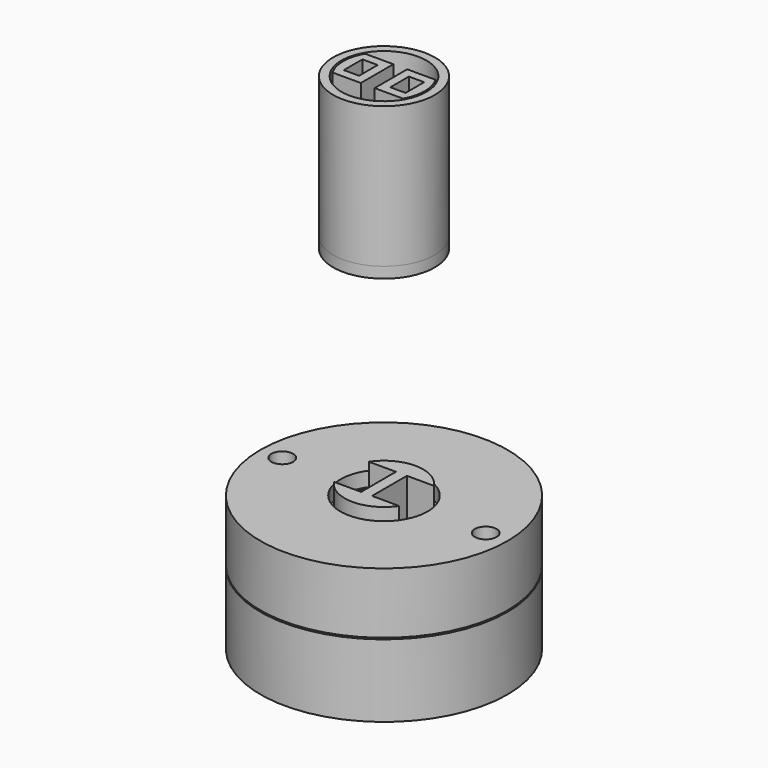
from build123d import *

# Parameters (mm, degrees)
F5_R      = 17
F5_W      = 21.213204
F5_H      = 21.213204
F5_R_2    = 8.1
F5_R_3    = 6
F6_DEPTH  = 0.5
F7_DEPTH  = 10
F8_W      = 20.78894
F8_H      = 20.78894
F8_R      = 6
F8_W_2    = 1.5
F8_H_2    = 8
F9_DEPTH  = 0.9
F10_W     = 20.364676
F10_H     = 20.364676
F10_R     = 8.1
F11_DEPTH = 8.6
F12_R     = 1.1
F12_R_2   = 1
F14_W     = 2
F14_H     = 15
F18_R     = 17
F18_W     = 21.213204
F18_H     = 21.213204
F18_R_2   = 8.2
F18_R_3   = 6
F19_DEPTH = 2
F20_DEPTH = 6.4
F21_R     = 1.5
F22_DEPTH = 18.6
F25_DEPTH = 18.4
F27_W     = 2.1
F27_H     = 3.2
F28_DEPTH = 1
F29_DEPTH = 19.4
F30_R     = 7
F30_R_2   = 5.85
F30_R_3   = 4
F31_DEPTH = 1.5
F32_DEPTH = 19.4
F34_DEPTH = 0.9


with BuildPart() as f6:
    # F5 (on Top) → F6 (new body)
    with BuildSketch(Plane.XY):
        Circle(F5_R)
        with BuildLine():
            ThreePointArc((10.606602, 10.606602), (13.858193, 5.740251), (15, 0))
            ThreePointArc((15, 0), (13.858193, -5.740251), (10.606602, -10.606602))
            ThreePointArc((10.606602, -10.606602), (0, -15), (-10.606602, -10.606602))
            ThreePointArc((-10.606602, -10.606602), (-15, 0), (-10.606602, 10.606602))
            ThreePointArc((-10.606602, 10.606602), (0, 15), (10.606602, 10.606602))
        make_face(mode=Mode.SUBTRACT)
        with BuildLine():
            Line((-10.606602, 10.606602), (10.606602, 10.606602))
            ThreePointArc((10.606602, 10.606602), (0, 15), (-10.606602, 10.606602))
        make_face()
        with BuildLine():
            Line((-10.606602, -10.606602), (-10.606602, 10.606602))
            ThreePointArc((-10.606602, 10.606602), (-15, 0), (-10.606602, -10.606602))
        make_face()
        with BuildLine():
            ThreePointArc((10.606602, -10.606602), (13.858193, -5.740251), (15, 0))
            ThreePointArc((15, 0), (13.858193, 5.740251), (10.606602, 10.606602))
            Line((10.606602, 10.606602), (10.606602, -10.606602))
        make_face()
        with BuildLine():
            ThreePointArc((-10.606602, -10.606602), (0, -15), (10.606602, -10.606602))
            Line((10.606602, -10.606602), (-10.606602, -10.606602))
        make_face()
        Rectangle(F5_W, F5_H)
        Circle(F5_R_2, mode=Mode.SUBTRACT)
        Circle(F5_R_2)
        Circle(F5_R_3, mode=Mode.SUBTRACT)
    extrude(amount=F6_DEPTH)

    # F5 (on Top) → F7 (join)
    with BuildSketch(Plane.XY):
        Circle(F5_R)
        with BuildLine():
            ThreePointArc((10.606602, 10.606602), (13.858193, 5.740251), (15, 0))
            ThreePointArc((15, 0), (13.858193, -5.740251), (10.606602, -10.606602))
            ThreePointArc((10.606602, -10.606602), (0, -15), (-10.606602, -10.606602))
            ThreePointArc((-10.606602, -10.606602), (-15, 0), (-10.606602, 10.606602))
            ThreePointArc((-10.606602, 10.606602), (0, 15), (10.606602, 10.606602))
        make_face(mode=Mode.SUBTRACT)
        with BuildLine():
            Line((-10.606602, -10.606602), (-10.606602, 10.606602))
            ThreePointArc((-10.606602, 10.606602), (-15, 0), (-10.606602, -10.606602))
        make_face()
        with BuildLine():
            Line((-10.606602, 10.606602), (10.606602, 10.606602))
            ThreePointArc((10.606602, 10.606602), (0, 15), (-10.606602, 10.606602))
        make_face()
        with BuildLine():
            ThreePointArc((10.606602, -10.606602), (13.858193, -5.740251), (15, 0))
            ThreePointArc((15, 0), (13.858193, 5.740251), (10.606602, 10.606602))
            Line((10.606602, 10.606602), (10.606602, -10.606602))
        make_face()
        with BuildLine():
            ThreePointArc((-10.606602, -10.606602), (0, -15), (10.606602, -10.606602))
            Line((10.606602, -10.606602), (-10.606602, -10.606602))
        make_face()
    extrude(amount=F7_DEPTH)


with BuildPart() as f9:
    # F8 (on face) → F9 (new body)
    with BuildSketch(Plane.XY.offset(0.5)):
        Rectangle(F8_W, F8_H)
        Circle(F8_R, mode=Mode.SUBTRACT)
        Circle(F8_R)
        Rectangle(F8_W_2, F8_H_2, mode=Mode.SUBTRACT)
    extrude(amount=F9_DEPTH)


with BuildPart() as f11:
    # F10 (on face) → F11 (new body)
    with BuildSketch(Plane.XY.offset(1.4)):
        Rectangle(F10_W, F10_H)
        Circle(F10_R, mode=Mode.SUBTRACT)
    extrude(amount=F11_DEPTH)

    # F12 (on Front) → F13 (revolve, cut)
    with BuildSketch(Plane.XZ):
        with Locations((8.5, 7.44)):
            Circle(F12_R)
        with Locations((8.5, 7.44)):
            Circle(F12_R_2, mode=Mode.SUBTRACT)
        with Locations((8.5, 4)):
            Circle(F12_R)
        with Locations((8.5, 4)):
            Circle(F12_R_2, mode=Mode.SUBTRACT)
        with Locations((8.5, 7.44)):
            Circle(F12_R_2)
        with Locations((8.5, 4)):
            Circle(F12_R_2)
    revolve(axis=Axis((0, 0, 11.757353), (0, 0, -1)), mode=Mode.SUBTRACT)


with BuildPart() as f15:
    # F14 (on Front) → F15 (revolve)
    with BuildSketch(Plane.XZ):
        with Locations((6.6, 9.1)):
            Rectangle(F14_W, F14_H)
    revolve(axis=Axis((0, 0, 5.77183), (0, 0, 1)))


with BuildPart() as f16:
    # F12 (on Front) → F16 (revolve)
    with BuildSketch(Plane.XZ):
        with Locations((8.5, 7.44)):
            Circle(F12_R_2)
    revolve(axis=Axis((0, 0, 11.757353), (0, 0, -1)))


with BuildPart() as f16b:
    # F12 (on Front) → F16, piece 2 (revolve)
    with BuildSketch(Plane.XZ):
        with Locations((8.5, 4)):
            Circle(F12_R_2)
    revolve(axis=Axis((0, 0, 11.757353), (0, 0, -1)))


with BuildPart() as f19:
    # F18 (on offset) → F19 (new body)
    with BuildSketch(Plane.XY.offset(16.6)):
        Circle(F18_R)
        with BuildLine():
            ThreePointArc((10.606602, 10.606602), (13.858193, 5.740251), (15, 0))
            ThreePointArc((15, 0), (13.858193, -5.740251), (10.606602, -10.606602))
            ThreePointArc((10.606602, -10.606602), (0, -15), (-10.606602, -10.606602))
            ThreePointArc((-10.606602, -10.606602), (-15, 0), (-10.606602, 10.606602))
            ThreePointArc((-10.606602, 10.606602), (0, 15), (10.606602, 10.606602))
        make_face(mode=Mode.SUBTRACT)
        Rectangle(F18_W, F18_H)
        Circle(F18_R_2, mode=Mode.SUBTRACT)
        Circle(F18_R_2)
        Circle(F18_R_3, mode=Mode.SUBTRACT)
        with BuildLine():
            Line((-10.606602, 10.606602), (10.606602, 10.606602))
            ThreePointArc((10.606602, 10.606602), (0, 15), (-10.606602, 10.606602))
        make_face()
        with BuildLine():
            Line((-10.606602, -10.606602), (-10.606602, 10.606602))
            ThreePointArc((-10.606602, 10.606602), (-15, 0), (-10.606602, -10.606602))
        make_face()
        with BuildLine():
            ThreePointArc((-10.606602, -10.606602), (0, -15), (10.606602, -10.606602))
            Line((10.606602, -10.606602), (-10.606602, -10.606602))
        make_face()
        with BuildLine():
            ThreePointArc((10.606602, -10.606602), (13.858193, -5.740251), (15, 0))
            ThreePointArc((15, 0), (13.858193, 5.740251), (10.606602, 10.606602))
            Line((10.606602, 10.606602), (10.606602, -10.606602))
        make_face()
    extrude(amount=F19_DEPTH)

    # F18 (on offset) → F20 (join)
    with BuildSketch(Plane.XY.offset(16.6)):
        Circle(F18_R)
        with BuildLine():
            ThreePointArc((10.606602, 10.606602), (13.858193, 5.740251), (15, 0))
            ThreePointArc((15, 0), (13.858193, -5.740251), (10.606602, -10.606602))
            ThreePointArc((10.606602, -10.606602), (0, -15), (-10.606602, -10.606602))
            ThreePointArc((-10.606602, -10.606602), (-15, 0), (-10.606602, 10.606602))
            ThreePointArc((-10.606602, 10.606602), (0, 15), (10.606602, 10.606602))
        make_face(mode=Mode.SUBTRACT)
        with BuildLine():
            ThreePointArc((-10.606602, -10.606602), (0, -15), (10.606602, -10.606602))
            Line((10.606602, -10.606602), (-10.606602, -10.606602))
        make_face()
        with BuildLine():
            Line((-10.606602, -10.606602), (-10.606602, 10.606602))
            ThreePointArc((-10.606602, 10.606602), (-15, 0), (-10.606602, -10.606602))
        make_face()
        with BuildLine():
            ThreePointArc((10.606602, -10.606602), (13.858193, -5.740251), (15, 0))
            ThreePointArc((15, 0), (13.858193, 5.740251), (10.606602, 10.606602))
            Line((10.606602, 10.606602), (10.606602, -10.606602))
        make_face()
        with BuildLine():
            Line((-10.606602, 10.606602), (10.606602, 10.606602))
            ThreePointArc((10.606602, 10.606602), (0, 15), (-10.606602, 10.606602))
        make_face()
    extrude(amount=-F20_DEPTH)


with BuildPart() as f22_tool:
    # F21 (on face) → F22 (new body, through all)
    with BuildSketch(Plane.XY.offset(18.6)):
        with Locations((-14, 0)):
            Circle(F21_R)
        with Locations((14, 0)):
            Circle(F21_R)
    extrude(amount=-F22_DEPTH)


with BuildPart() as f6_1:
    add(f6.part)

    # F22: cut by f22_tool
    add(f22_tool.part, mode=Mode.SUBTRACT)


with BuildPart() as f19_1:
    add(f19.part)

    # F22: cut by f22_tool
    add(f22_tool.part, mode=Mode.SUBTRACT)


with BuildPart() as f25:
    # F24 (on offset) → F25 (new body, through all)
    with BuildSketch(Plane.XY.offset(20)):
        with BuildLine():
            Line((-0.75, -3), (-4.489989, -3))
            ThreePointArc((-4.489989, -3), (0, -5.4), (4.489989, -3))
            Line((4.489989, -3), (0.75, -3))
            Line((0.75, -3), (0.75, 0))
            Line((0.75, 0), (0.75, 3))
            Line((0.75, 3), (4.489989, 3))
            ThreePointArc((4.489989, 3), (0, 5.4), (-4.489989, 3))
            Line((-4.489989, 3), (-0.75, 3))
            Line((-0.75, 3), (-0.75, 0))
            Line((-0.75, 0), (-0.75, -3))
        make_face()
    extrude(amount=-F25_DEPTH)


with BuildPart() as f28:
    # F27 (on offset) → F28 (new body)
    with BuildSketch(Plane.XY.offset(50)):
        with BuildLine():
            Line((0.95, 2.8), (4.849742, 2.8))
            ThreePointArc((4.849742, 2.8), (0, 5.6), (-4.849742, 2.8))
            Line((-4.849742, 2.8), (-0.95, 2.8))
            Line((-0.95, 2.8), (-0.95, -2.8))
            Line((-0.95, -2.8), (-4.849742, -2.8))
            ThreePointArc((-4.849742, -2.8), (0, -5.6), (4.849742, -2.8))
            Line((4.849742, -2.8), (0.95, -2.8))
            Line((0.95, -2.8), (0.95, 2.8))
        make_face()
        with BuildLine():
            ThreePointArc((4.849742, -2.8), (5.409185, -1.449387), (5.6, 0))
            ThreePointArc((5.6, 0), (5.409185, 1.449387), (4.849742, 2.8))
            Line((4.849742, 2.8), (0.95, 2.8))
            Line((0.95, 2.8), (0.95, -2.8))
            Line((0.95, -2.8), (4.849742, -2.8))
        make_face()
        with Locations((3.2, 0)):
            Rectangle(F27_W, F27_H, mode=Mode.SUBTRACT)
        with BuildLine():
            Line((-0.95, 2.8), (-4.849742, 2.8))
            ThreePointArc((-4.849742, 2.8), (-5.6, 0), (-4.849742, -2.8))
            Line((-4.849742, -2.8), (-0.95, -2.8))
            Line((-0.95, -2.8), (-0.95, 2.8))
        make_face()
        with Locations((-3.2, 0)):
            Rectangle(F27_W, F27_H, mode=Mode.SUBTRACT)
        with Locations((3.2, 0)):
            Rectangle(F27_W, F27_H)
        with Locations((-3.2, 0)):
            Rectangle(F27_W, F27_H)
    extrude(amount=F28_DEPTH)

    # F27 (on offset) → F29 (join)
    with BuildSketch(Plane.XY.offset(50)):
        with BuildLine():
            Line((-0.95, 2.8), (-4.849742, 2.8))
            ThreePointArc((-4.849742, 2.8), (-5.6, 0), (-4.849742, -2.8))
            Line((-4.849742, -2.8), (-0.95, -2.8))
            Line((-0.95, -2.8), (-0.95, 2.8))
        make_face()
        with Locations((-3.2, 0)):
            Rectangle(F27_W, F27_H, mode=Mode.SUBTRACT)
        with BuildLine():
            ThreePointArc((4.849742, -2.8), (5.409185, -1.449387), (5.6, 0))
            ThreePointArc((5.6, 0), (5.409185, 1.449387), (4.849742, 2.8))
            Line((4.849742, 2.8), (0.95, 2.8))
            Line((0.95, 2.8), (0.95, -2.8))
            Line((0.95, -2.8), (4.849742, -2.8))
        make_face()
        with Locations((3.2, 0)):
            Rectangle(F27_W, F27_H, mode=Mode.SUBTRACT)
    extrude(amount=F29_DEPTH)


with BuildPart() as f31:
    # F30 (on offset) → F31 (new body)
    with BuildSketch(Plane.XY.offset(50)):
        Circle(F30_R)
        Circle(F30_R_2, mode=Mode.SUBTRACT)
        Circle(F30_R_2)
        Circle(F30_R_3, mode=Mode.SUBTRACT)
    extrude(amount=-F31_DEPTH)

    # F30 (on offset) → F32 (join)
    with BuildSketch(Plane.XY.offset(50)):
        Circle(F30_R)
        Circle(F30_R_2, mode=Mode.SUBTRACT)
    extrude(amount=F32_DEPTH)


with BuildPart() as f34:
    # F33 (on face) → F34 (new body)
    with BuildSketch(Plane.XY.offset(1.4)):
        Polygon((-0.75, 4), (-0.75, 10.39447), (-10.39447, 10.39447), (-10.39447, -10.39447), (-0.75, -10.39447), (-0.75, -4), align=None)
    extrude(amount=F34_DEPTH)


with BuildPart() as f34b:
    # F33 (on face) → F34, piece 2 (new body)
    with BuildSketch(Plane.XY.offset(1.4)):
        Polygon((10.39447, 10.39447), (0.75, 10.39447), (0.75, 4), (0.75, -4), (0.75, -10.39447), (10.39447, -10.39447), align=None)
    extrude(amount=F34_DEPTH)


solid = Compound([f9.part, f11.part, f15.part, f16.part, f16b.part, f6_1.part, f19_1.part, f25.part, f28.part, f31.part, f34.part, f34b.part])
